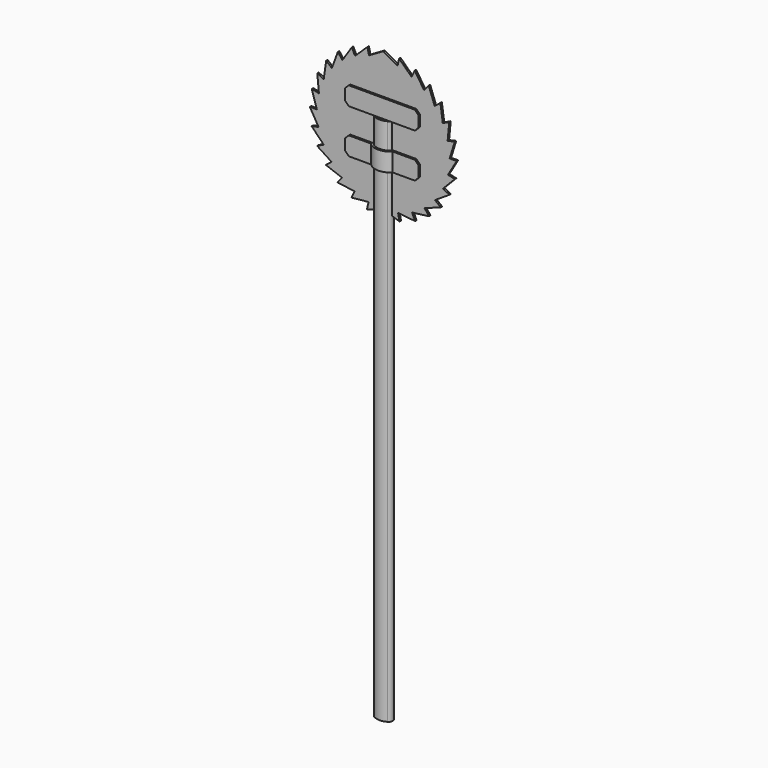
from build123d import *

# Parameters (mm, degrees)
F1_DEPTH      = 914.4
F3_DEPTH      = 1.5875
F3_DEPTH_BACK = 1.5875
F5_DEPTH      = 4.7752
F5_DEPTH_BACK = 4.7752
F7_DEPTH      = 4.7752
F7_DEPTH_BACK = 4.7752
F9_START      = 838.2
F9_DEPTH      = 31.75
F10_R         = 7.62


with BuildPart() as f1:
    # F0 (on Top) → F1 (new body)
    with BuildSketch(Plane.XY):
        with BuildLine():
            ThreePointArc((-19.05, 0), (0, -9.525), (19.05, 0))
            ThreePointArc((19.05, 0), (0, 9.525), (-19.05, 0))
        make_face()
    extrude(amount=F1_DEPTH)

    # F10
    f10_edges = [f1.edges().sort_by_distance(p)[0] for p in [
        (19.05, 0, 457.2),
        (-19.05, 0, 457.2),
    ]]
    fillet(f10_edges, radius=F10_R)


with BuildPart() as f3:
    # F2 (on Front) → F3 (new body, two sides)
    with BuildSketch(Plane.XZ) as f3_sk:
        Polygon((111.9438048034, 863.6422354789), (126.9993189541, 889.4159148914), (114.8417657116, 889.3760996587), (123.6705603008, 917.8893148914), (111.3035042707, 915.0003834023), (114.1262108525, 944.7154197367), (102.9643832521, 939.2663129528), (98.7810034847, 968.8205070803), (88.9029031363, 960.8384563722), (78.515398819, 988.8215014328), (70.6638589371, 978.8393512895), (54.3031673817, 1003.8049041301), (48.8728506435, 992.3244137171), (27.361352482, 1013.0175648461), (24.7180633611, 1001.0366410167), (1.1008259294, 1014.7136328074), (0, 1015.351132737), (-1.1008259294, 1014.7136328074), (-24.7180633611, 1001.0366410167), (-27.361352482, 1013.0175648461), (-48.8728506435, 992.3244137171), (-54.3031673817, 1003.8049041301), (-70.6638589371, 978.8393512895), (-78.515398819, 988.8215014328), (-88.9029031363, 960.8384563722), (-98.7810034847, 968.8205070803), (-102.9643832521, 939.2663129528), (-114.1262108525, 944.7154197367), (-111.3035042707, 915.0003834023), (-123.6705603008, 917.8893148914), (-114.8417657116, 889.3760996587), (-126.9993189541, 889.4159148914), (-111.9438048034, 863.6422354789), (-123.8619292978, 860.9425148914), (-103.0482818511, 839.5475823894), (-114.4980909457, 834.0528693216), (-89.441039496, 817.8326587972), (-99.3789327734, 809.9251764414), (-71.3379860484, 799.6950071577), (-79.2644289427, 789.7722301753), (-49.6490830757, 786.0463281386), (-55.1656478619, 774.6070312651), (-25.4645371669, 777.572681326), (-28.2939301854, 765.19186814), (0, 774.7), (28.2939301854, 765.19186814), (25.4645371669, 777.572681326), (55.1656478619, 774.6070312651), (49.6490830757, 786.0463281386), (79.2644289427, 789.7722301753), (71.3379860484, 799.6950071577), (99.3789327734, 809.9251764414), (89.441039496, 817.8326587972), (114.4980909457, 834.0528693216), (103.0482818511, 839.5475823894), (123.8619292978, 860.9425148914), align=None)
    extrude(amount=F3_DEPTH)
    extrude(f3_sk.sketch, amount=-F3_DEPTH_BACK)

    # F6 (on Front) → F7 (join, two sides)
    with BuildSketch(Plane.XZ) as f7_sk:
        Polygon((-57.15, 838.2), (57.15, 838.2), (63.5, 844.55), (63.5, 863.6), (57.15, 869.95), (-57.15, 869.95), (-63.5, 863.6), (-63.5, 844.55), align=None)
    extrude(amount=F7_DEPTH)
    extrude(f7_sk.sketch, amount=-F7_DEPTH_BACK)

    # F8 (on Top) → F9 (join)
    with BuildSketch(Plane.XY.offset(F9_START)):
        with BuildLine():
            ThreePointArc((-22.225, 0), (0, -12.7), (22.225, 0))
            ThreePointArc((22.225, 0), (0, 12.7), (-22.225, 0))
        make_face()
    extrude(amount=F9_DEPTH)


with BuildPart() as f5:
    # F4 (on Front) → F5 (new body, two sides)
    with BuildSketch(Plane.XZ) as f5_sk:
        Polygon((-57.15, 914.4), (57.15, 914.4), (63.5, 920.75), (63.5, 939.8), (57.15, 946.15), (-57.15, 946.15), (-63.5, 939.8), (-63.5, 920.75), align=None)
    extrude(amount=F5_DEPTH)
    extrude(f5_sk.sketch, amount=-F5_DEPTH_BACK)


solid = Compound([f1.part, f3.part, f5.part])
